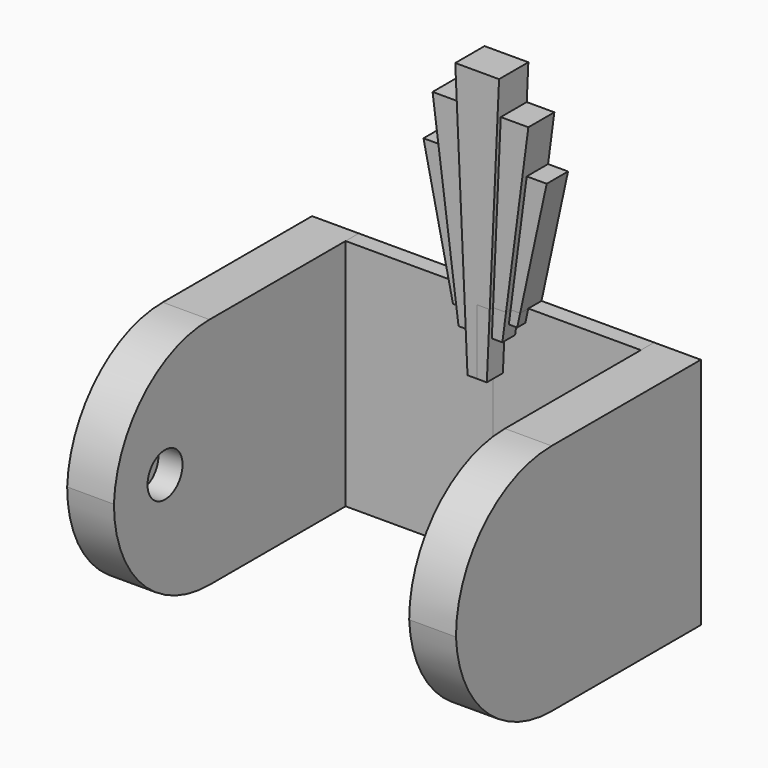
from build123d import *

# Parameters (mm, degrees)
F0_W         = 431.6743224388
F0_H         = 2155.444
F1_DEPTH     = 2825.242
F0_W_2       = 1362.583
F2_DEPTH     = 152.4
F3_R         = 1103.778440717
F4_T1_DEPTH  = 5944.4309410994
F6_DEPTH     = 337.82
F7_DEPTH     = 337.82
F8_DEPTH     = 299.72
F9_DEPTH     = 299.72
F10_DEPTH    = 299.72
F11_DEPTH    = 299.72
F12_DEPTH    = 246.38
F13_DEPTH    = 246.38
F14_DEPTH    = 246.38
F15_DEPTH    = 246.38
F16_DEPTH    = 152.4
F17_DEPTH    = 2825.242
F18_R        = 1103.7824
F19_T1_DEPTH = 5944.4300053009
F20_R        = 201.8308928609
F21_DEPTH    = 222
F22_DEPTH    = 2969


# Not quite as in the source:
# - a fillet or chamfer that OpenCascade refuses, or shapes differently, is made with other operations: its cross-section is extruded or revolved along the edge and cut away or added


with BuildPart() as f1:
    # F0 (on Front) → F1 (new body)
    with BuildSketch(Plane.XZ):
        with Locations((-1578.4201612194, 95.021261747)):
            Rectangle(F0_W, F0_H)
    extrude(amount=F1_DEPTH)

    # F3
    f3_edges = [f1.edges().sort_by_distance(p)[0] for p in [
        (-1578.420161, -2825.242, -982.700738),
    ]]
    fillet(f3_edges, radius=F3_R)

    # F4: fillet of radius 1103.7824 on 1 edges, made by hand

    # F4_s2 → F4_t1 (cut)
    with BuildSketch(Plane.YZ.offset(-4550.6356317691)):
        with BuildLine():
            ThreePointArc((-2825.242, 121.077702464), (-2484.5338146575, 867.6664514598), (-1722.6906762679, 1172.743261747))
            Line((-1722.6906762679, 1172.743261747), (-2825.242, 1172.743261747))
            Line((-2825.242, 1172.743261747), (-2825.242, 121.077702464))
        make_face()
    extrude(amount=F4_T1_DEPTH, mode=Mode.SUBTRACT)

    # F20 (on face) → F21 (cut)
    with BuildSketch(Plane.YZ.offset(-1362.583)):
        with Locations((-2235.8012199402, 121.077702464)):
            Circle(F20_R)
    extrude(amount=-F21_DEPTH, mode=Mode.SUBTRACT)


with BuildPart() as f2:
    # F0 (on Front) → F2 (new body)
    with BuildSketch(Plane.XZ):
        with Locations((681.2915, 95.021261747)):
            Rectangle(F0_W_2, F0_H)
    extrude(amount=F2_DEPTH)


with BuildPart() as f6:
    # F5 (on face) → F6 (new body)
    with BuildSketch(Plane(origin=(0, 0, 0), x_dir=(-1, 0, 0), z_dir=(0, 1, 0))):
        Polygon((202.1480798721, 3072.124004364), (0, 3072.124004364), (-202.1480798721, 3072.124004364), (-187.3023343028, 2743.8715661091), (-116.2455245279, 1172.743261747), (0, 1172.743261747), (0, 571.585059166), (89.0571759208, 571.585059166), (104.7298349479, 918.121278286), (187.3023343028, 2743.8715661091), align=None)
    extrude(amount=-F6_DEPTH)


with BuildPart() as f7:
    # F5 (on face) → F7 (new body)
    with BuildSketch(Plane(origin=(0, 0, 0), x_dir=(-1, 0, 0), z_dir=(0, 1, 0))):
        Polygon((0, 1172.743261747), (-116.2455245279, 1172.743261747), (-104.7298349479, 918.121278286), (-89.0571759208, 571.585059166), (0, 571.585059166), align=None)
    extrude(amount=-F7_DEPTH)


with BuildPart() as f8:
    # F5 (on face) → F8 (new body)
    with BuildSketch(Plane(origin=(0, 0, 0), x_dir=(-1, 0, 0), z_dir=(0, 1, 0))):
        Polygon((-116.2455245279, 1172.743261747), (-187.3023343028, 2743.8715661091), (-442.0145153999, 2743.8715661091), (-384.2649371563, 2304.3089867597), (-235.6002271823, 1172.743261747), align=None)
    extrude(amount=-F8_DEPTH)


with BuildPart() as f9:
    # F5 (on face) → F9 (new body)
    with BuildSketch(Plane(origin=(0, 0, 0), x_dir=(-1, 0, 0), z_dir=(0, 1, 0))):
        Polygon((-104.7298349479, 918.121278286), (-116.2455245279, 1172.743261747), (-235.6002271823, 1172.743261747), (-219.1109658235, 1047.2347736359), (-202.1480798721, 918.121278286), align=None)
    extrude(amount=-F9_DEPTH)


with BuildPart() as f10:
    # F5 (on face) → F10 (new body)
    with BuildSketch(Plane(origin=(0, 0, 0), x_dir=(-1, 0, 0), z_dir=(0, 1, 0))):
        Polygon((442.0145153999, 2743.8715661091), (187.3023343028, 2743.8715661091), (104.7298349479, 918.121278286), (202.1480798721, 918.121278286), (219.1109658235, 1047.2347736359), (384.2649371563, 2304.3089867597), align=None)
    extrude(amount=-F10_DEPTH)


with BuildPart() as f11:
    # F5 (on face) → F11 (new body)
    with BuildSketch(Plane(origin=(0, 0, 0), x_dir=(-1, 0, 0), z_dir=(0, 1, 0))):
        Polygon((442.0145153999, 2743.8715661091), (187.3023343028, 2743.8715661091), (104.7298349479, 918.121278286), (202.1480798721, 918.121278286), (219.1109658235, 1047.2347736359), (384.2649371563, 2304.3089867597), align=None)
    extrude(amount=-F11_DEPTH)


with BuildPart() as f12:
    # F5 (on face) → F12 (new body)
    with BuildSketch(Plane(origin=(0, 0, 0), x_dir=(-1, 0, 0), z_dir=(0, 1, 0))):
        Polygon((-323.5727009185, 1172.743261747), (-235.6002271823, 1172.743261747), (-384.2649371563, 2304.3089867597), (-568.5825943947, 2304.3089867597), align=None)
    extrude(amount=-F12_DEPTH)


with BuildPart() as f13:
    # F5 (on face) → F13 (new body)
    with BuildSketch(Plane(origin=(0, 0, 0), x_dir=(-1, 0, 0), z_dir=(0, 1, 0))):
        Polygon((-219.1109658235, 1047.2347736359), (-235.6002271823, 1172.743261747), (-323.5727009185, 1172.743261747), (-296.3972389698, 1047.2347736359), align=None)
    extrude(amount=-F13_DEPTH)


with BuildPart() as f14:
    # F5 (on face) → F14 (new body)
    with BuildSketch(Plane(origin=(0, 0, 0), x_dir=(-1, 0, 0), z_dir=(0, 1, 0))):
        Polygon((568.5825943947, 2304.3089867597), (384.2649371563, 2304.3089867597), (219.1109658235, 1047.2347736359), (296.3972389698, 1047.2347736359), align=None)
    extrude(amount=-F14_DEPTH)


with BuildPart() as f15:
    # F5 (on face) → F15 (new body)
    with BuildSketch(Plane(origin=(0, 0, 0), x_dir=(-1, 0, 0), z_dir=(0, 1, 0))):
        Polygon((568.5825943947, 2304.3089867597), (384.2649371563, 2304.3089867597), (219.1109658235, 1047.2347736359), (296.3972389698, 1047.2347736359), align=None)
    extrude(amount=-F15_DEPTH)


with BuildPart() as f16:
    # F0 (on Front) → F16 (new body)
    with BuildSketch(Plane.XZ):
        with Locations((-681.2915, 95.021261747)):
            Rectangle(F0_W_2, F0_H)
    extrude(amount=F16_DEPTH)


with BuildPart() as f17:
    # F0 (on Front) → F17 (new body)
    with BuildSketch(Plane.XZ):
        with Locations((1578.4201612194, 95.021261747)):
            Rectangle(F0_W, F0_H)
    extrude(amount=F17_DEPTH)

    # F18
    f18_edges = [f17.edges().sort_by_distance(p)[0] for p in [
        (1578.420161, -2825.242, 1172.743262),
    ]]
    fillet(f18_edges, radius=F18_R)

    # F19: fillet of radius 1103.7824 on 1 edges, made by hand

    # F19_s2 → F19_t1 (cut)
    with BuildSketch(Plane.YZ.offset(-1393.794841431)):
        with BuildLine():
            ThreePointArc((-2825.242, 68.960861747), (-2484.5325677323, -677.6252958612), (-1722.6908634276, -982.700738253))
            Line((-1722.6908634276, -982.700738253), (-2825.242, -982.700738253))
            Line((-2825.242, -982.700738253), (-2825.242, 68.960861747))
        make_face()
    extrude(amount=F19_T1_DEPTH, mode=Mode.SUBTRACT)

    # F20 (on face) → F22 (cut)
    with BuildSketch(Plane.YZ.offset(-1362.583)):
        with Locations((-2235.8012199402, 121.077702464)):
            Circle(F20_R)
    extrude(amount=F22_DEPTH, mode=Mode.SUBTRACT)


solid = Compound([f1.part, f2.part, f6.part, f7.part, f8.part, f9.part, f10.part, f11.part, f12.part, f13.part, f14.part, f15.part, f16.part, f17.part])
